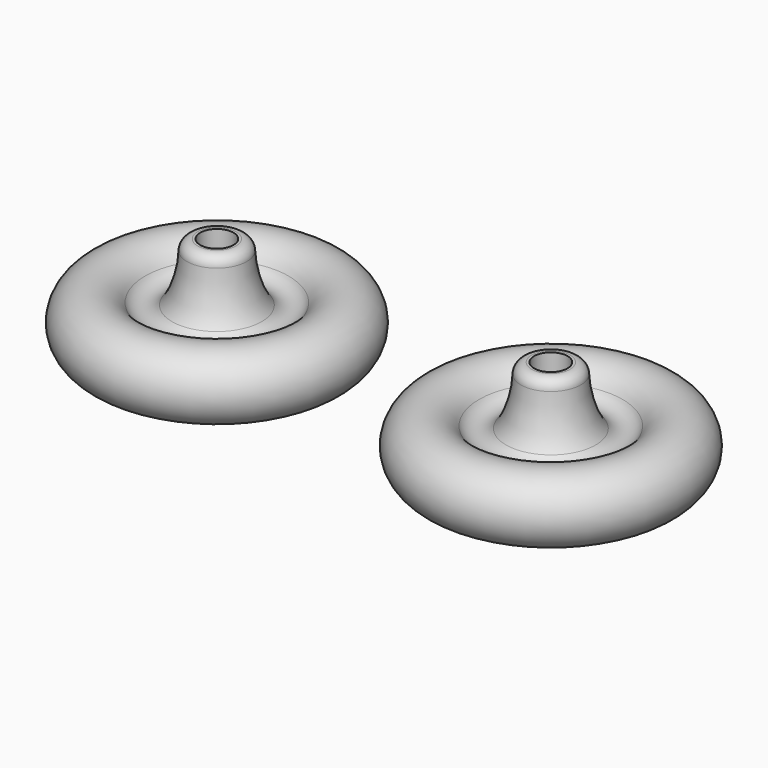
from build123d import *


with BuildPart() as f1:
    # F0 (on Front) → F1 (revolve)
    with BuildSketch(Plane.XZ):
        with BuildLine():
            add(Edge.make_bspline(
                [(0, -27.94), (-0.6298177026, -24.4216997861), (-1.7059942815, -18.140745574), (-7.5123536473, -16.3480573189), (-10.2070122078, -15.7636512276)],
                knots=[0, 0, 0, 0, 0.495905004, 0.8775780379, 0.8775780379, 0.8775780379, 0.8775780379], degree=3))
            Line((0, -27.94), (0, -12.7))
            Line((0, -12.7), (-3.175, -12.7))
            Line((-3.175, -12.7), (-3.175, 0))
            Line((-3.175, 0), (-3.6600066881, 0))
            ThreePointArc((-3.6600066881, 0), (-5.0677166308, -0.5666069752), (-5.6903692186, -1.9504402391))
            add(Edge.make_bspline(
                [(-5.6903692186, -1.9504402391), (-5.8378361062, -5.6215059664), (-7.0589469217, -9.3272503933), (-8.4991875523, -11.0362365317), (-8.5366888176, -11.0792262447)],
                knots=[0.0914542107, 0.0914542107, 0.0914542107, 0.0914542107, 0.6066753324, 0.6203805412, 0.6203805412, 0.6203805412, 0.6203805412], degree=3))
            ThreePointArc((-8.5366888176, -11.0792262447), (-11.1947209076, -12.1559778646), (-13.6361877206, -10.6513953831))
            ThreePointArc((-13.6361877206, -10.6513953831), (-25.3999207527, -14.0017243463), (-13.6032991556, -17.2343452501))
            ThreePointArc((-13.6032991556, -17.2343452501), (-12.141608162, -15.9529563971), (-10.2070122078, -15.7636512276))
        make_face()
    revolve(axis=Axis((0, 0, -20.32), (0, 0, 1)))


with BuildPart() as f2_1:
    # F2: copy of F1
    add(f1.part.moved(Location((63.5, 0, 0))))


solid = Compound([f1.part, f2_1.part])
